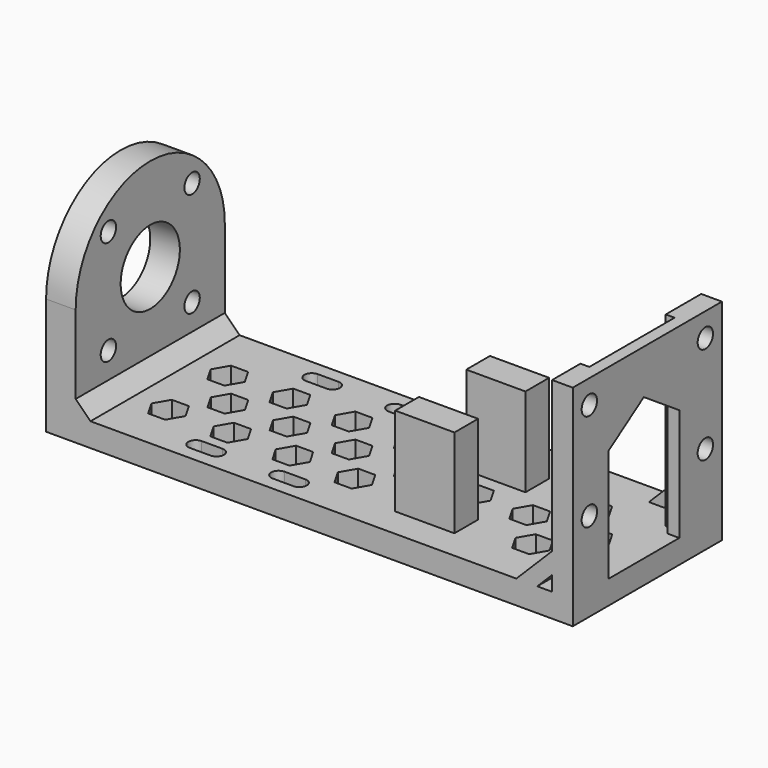
from build123d import *

# Parameters (mm, degrees)
F1_DEPTH  = 8
F2_R      = 3.25
F2_R_2    = 12.5
F3_DEPTH  = 10
F4_W      = 20
F4_H      = 10
F5_DEPTH  = 30
F7_DEPTH  = 63
F9_DEPTH  = 4
F11_DEPTH = 7
F13_D     = 6.5
F13_DEPTH = 15
F13_TIP   = 1.9527970118
F15_DEPTH = 63
F17_DEPTH = 8
F19_DEPTH = 8


# Not quite as in the source:
# - a pattern or mirror of a feature is missing from the dataset's text; its kind, count and spacing are read off the source's solid


with BuildPart() as f1:
    # F0 (on Top) → F1 (new body)
    with BuildSketch(Plane.XY):
        Polygon((76.5, 31.5), (-76.5, 31.5), (-76.5, -31.5), (76.5, -31.5), (101.5, -31.5), (101.5, 31.5), align=None)
    extrude(amount=F1_DEPTH)

    # F2 (on face) → F3 (join)
    with BuildSketch(Plane(origin=(-76.5, 0, 0), x_dir=(0, -1, 0), z_dir=(-1, 0, 0))):
        with BuildLine():
            Line((31.5, 8), (31.5, 39.5))
            ThreePointArc((31.5, 39.5), (0, 71), (-31.5, 39.5))
            Line((-31.5, 39.5), (-31.5, 8))
            Line((-31.5, 8), (31.5, 8))
        make_face()
        with Locations((-17.6776695297, 21.8223304703)):
            Circle(F2_R, mode=Mode.SUBTRACT)
        with Locations((17.6776695297, 21.8223304703)):
            Circle(F2_R, mode=Mode.SUBTRACT)
        with Locations((0, 39.5)):
            Circle(F2_R_2, mode=Mode.SUBTRACT)
        with Locations((-17.6776695297, 57.1776695297)):
            Circle(F2_R, mode=Mode.SUBTRACT)
        with Locations((17.6776695297, 57.1776695297)):
            Circle(F2_R, mode=Mode.SUBTRACT)
    extrude(amount=-F3_DEPTH)

    # F4 (on face) → F5 (join)
    with BuildSketch(Plane.XY.offset(8)):
        with Locations((43.5, 13.5)):
            Rectangle(F4_W, F4_H)
        with Locations((43.5, -16.5)):
            Rectangle(F4_W, F4_H)
    extrude(amount=F5_DEPTH)

    # F6 (on face) → F7 (join)
    with BuildSketch(Plane.XY.offset(8)):
        Polygon((97.5, 13.5), (101.5, 13.5), (101.5, 31.5), (94.5, 31.5), (94.5, 16.5), (97.5, 16.5), align=None)
        Polygon((94.5, -31.5), (101.5, -31.5), (101.5, -16.5), (97.5, -16.5), (97.5, -19.5), (94.5, -19.5), align=None)
    extrude(amount=F7_DEPTH)

    # F8 (on face) → F9 (join, through all)
    with BuildSketch(Plane.YZ.offset(101.5)):
        Polygon((13.5, 71), (-16.5, 71), (-16.5, 46), (-1.5, 56), (13.5, 46), align=None)
    extrude(amount=-F9_DEPTH)

    # F10 (on face) → F11 (join)
    with BuildSketch(Plane.XZ.offset(31.5)):
        Polygon((89.5, 8), (94.5, 13), (94.5, 20.0710678119), (85.9644660941, 11.5355339059), (82.4289321881, 8), align=None)
    f11 = extrude(amount=-F11_DEPTH)

    # F11_copies: F11 across plane
    add(f11.mirror(Plane.ZX))

    # F13
    with Locations(Plane.YZ.offset(101.5)):
        with Locations((-24.5, 63), (24.5, 63), (24.5, 30), (-24.5, 30)):
            Hole(F13_D / 2, depth=F13_DEPTH)
            with Locations((0, 0, -(F13_DEPTH + F13_TIP / 2))):  # 118° drill point
                Cone(0, F13_D / 2, F13_TIP, mode=Mode.SUBTRACT)

    # F14 (on face) → F15 (join)
    with BuildSketch(Plane.XZ.offset(31.5)):
        Polygon((-66.5, 13), (-66.5, 8), (-61.5, 8), align=None)
    extrude(amount=-F15_DEPTH)

    # F16 (on face) → F17 (cut)
    with BuildSketch(Plane.XY.offset(8)):
        with BuildLine():
            ThreePointArc((-24.5, 22), (-22, 24.5), (-24.5, 27))
            Line((-24.5, 27), (-31.5, 27))
            ThreePointArc((-31.5, 27), (-34, 24.5), (-31.5, 22))
            Line((-31.5, 22), (-24.5, 22))
        make_face()
        with BuildLine():
            ThreePointArc((3.5, 22), (6, 24.5), (3.5, 27))
            Line((3.5, 27), (-3.5, 27))
            ThreePointArc((-3.5, 27), (-6, 24.5), (-3.5, 22))
            Line((-3.5, 22), (3.5, 22))
        make_face()
        with BuildLine():
            ThreePointArc((3.5, -27), (6, -24.5), (3.5, -22))
            Line((3.5, -22), (-3.5, -22))
            ThreePointArc((-3.5, -22), (-6, -24.5), (-3.5, -27))
            Line((-3.5, -27), (3.5, -27))
        make_face()
        with BuildLine():
            ThreePointArc((-24.5, -27), (-22, -24.5), (-24.5, -22))
            Line((-24.5, -22), (-31.5, -22))
            ThreePointArc((-31.5, -22), (-34, -24.5), (-31.5, -27))
            Line((-31.5, -27), (-24.5, -27))
        make_face()
    extrude(amount=-F17_DEPTH, mode=Mode.SUBTRACT)

    # F18 (on face) → F19 (cut)
    with BuildSketch(Plane.XY.offset(8)):
        Polygon((-49.5, 16.5), (-52.3867513459, 16.5), (-55.2735026919, 11.5), (-49.5, 11.5), align=None)
        Polygon((-46.6132486541, 16.5), (-49.5, 16.5), (-49.5, 11.5), (-55.2735026919, 11.5), (-52.3867513459, 6.5), (-46.6132486541, 6.5), (-43.7264973081, 11.5), align=None)
        Polygon((-42.3724755983, 4.0214471492), (-45.2592269442, -0.9785528508), (-42.3724755983, -5.9785528508), (-36.5989729064, -5.9785528508), (-33.7122215604, -0.9785528508), (-36.5989729064, 4.0214471492), align=None)
        Polygon((-31.3867513459, 16.5), (-34.2735026919, 11.5), (-31.3867513459, 6.5), (-25.6132486541, 6.5), (-22.7264973081, 11.5), (-25.6132486541, 16.5), align=None)
        Polygon((-21.3724755983, 4.0214471492), (-24.2592269442, -0.9785528508), (-21.3724755983, -5.9785528508), (-15.5989729064, -5.9785528508), (-12.7122215604, -0.9785528508), (-15.5989729064, 4.0214471492), align=None)
        Polygon((-10.3867513459, 16.5), (-13.2735026919, 11.5), (-10.3867513459, 6.5), (-4.6132486541, 6.5), (-1.7264973081, 11.5), (-4.6132486541, 16.5), align=None)
        Polygon((-0.3724755983, 4.0214471492), (-3.2592269442, -0.9785528508), (-0.3724755983, -5.9785528508), (5.4010270936, -5.9785528508), (8.2877784396, -0.9785528508), (5.4010270936, 4.0214471492), align=None)
        Polygon((10.6132486541, 16.5), (7.7264973081, 11.5), (10.6132486541, 6.5), (16.3867513459, 6.5), (19.2735026919, 11.5), (16.3867513459, 16.5), align=None)
        Polygon((20.6275244017, 4.0214471492), (17.7407730558, -0.9785528508), (20.6275244017, -5.9785528508), (26.4010270936, -5.9785528508), (29.2877784396, -0.9785528508), (26.4010270936, 4.0214471492), align=None)
        Polygon((-52.4131430724, -8.4999860695), (-55.2998944183, -13.4999860695), (-52.4131430724, -18.4999860695), (-46.6396403805, -18.4999860695), (-43.7528890345, -13.4999860695), (-46.6396403805, -8.4999860695), align=None)
        Polygon((-31.4131430724, -8.4999860695), (-34.2998944183, -13.4999860695), (-31.4131430724, -18.4999860695), (-25.6396403805, -18.4999860695), (-22.7528890345, -13.4999860695), (-25.6396403805, -8.4999860695), align=None)
        Polygon((-10.4131430724, -8.4999860695), (-13.2998944183, -13.4999860695), (-10.4131430724, -18.4999860695), (-4.6396403805, -18.4999860695), (-1.7528890345, -13.4999860695), (-4.6396403805, -8.4999860695), align=None)
        Polygon((10.5868569276, -8.4999860695), (7.7001055817, -13.4999860695), (10.5868569276, -18.4999860695), (16.3603596195, -18.4999860695), (19.2471109655, -13.4999860695), (16.3603596195, -8.4999860695), align=None)
        Polygon((77.7407730558, -0.9785528508), (80.6275244017, -5.9785528508), (86.4010270936, -5.9785528508), (89.2877784396, -0.9785528508), (86.4010270936, 4.0214471492), (80.6275244017, 4.0214471492), align=None)
        Polygon((79.2471109655, -13.4999860695), (76.3603596195, -8.4999860695), (70.5868569276, -8.4999860695), (67.7001055817, -13.4999860695), (70.5868569276, -18.4999860695), (76.3603596195, -18.4999860695), align=None)
        Polygon((76.3867513459, 16.5), (70.6132486541, 16.5), (67.7264973081, 11.5), (70.6132486541, 6.5), (76.3867513459, 6.5), (79.2735026919, 11.5), align=None)
        Polygon((68.2877784396, -0.9785528508), (65.4010270936, 4.0214471492), (59.6275244017, 4.0214471492), (56.7407730558, -0.9785528508), (59.6275244017, -5.9785528508), (65.4010270936, -5.9785528508), align=None)
        Polygon((37.7407730558, -0.9785528508), (40.6275244017, -5.9785528508), (46.4010270936, -5.9785528508), (49.2877784396, -0.9785528508), (46.4010270936, 4.0214471492), (40.6275244017, 4.0214471492), align=None)
    extrude(amount=-F19_DEPTH, mode=Mode.SUBTRACT)


solid = f1.part
